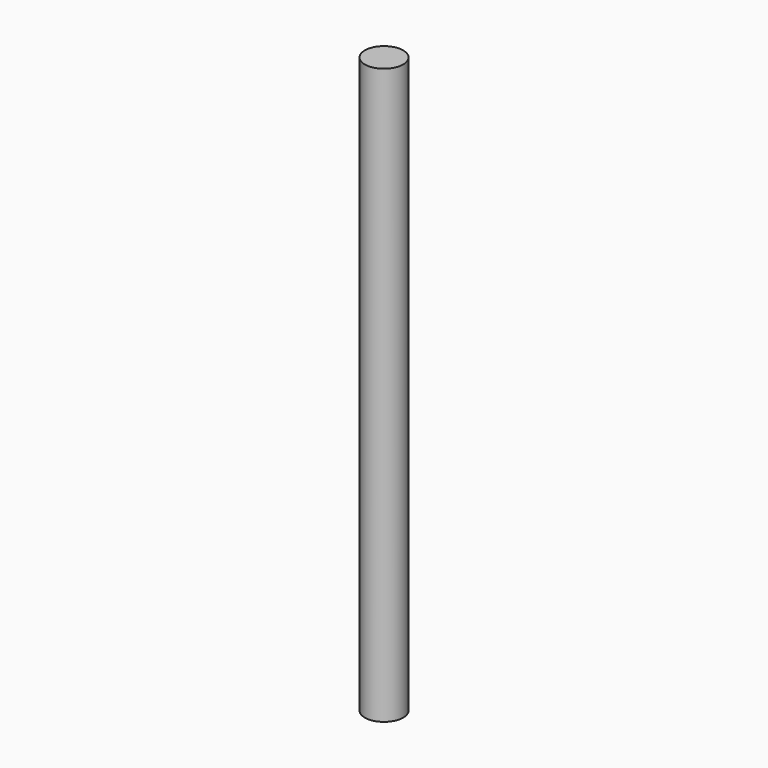
from build123d import *

# Parameters (mm, degrees)
F2_R          = 12.7
F3_DEPTH      = 266.7
F3_DEPTH_BACK = 114.3


# Not quite as in the source:
# - a variable given as a bare number and used for a length is read in inches; the dataset says mm whatever the document's units were


with BuildPart() as f3:
    # F2 (on Top) → F3 (new body, two sides)
    with BuildSketch(Plane.XY) as f3_sk:
        Circle(F2_R)
    extrude(amount=F3_DEPTH)
    extrude(f3_sk.sketch, amount=-F3_DEPTH_BACK)


solid = f3.part
